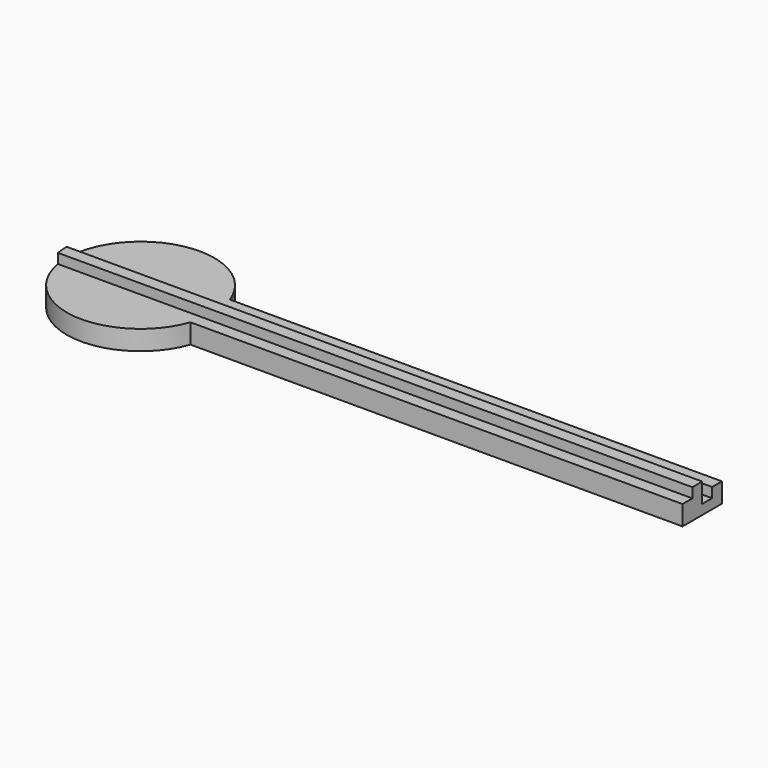
from build123d import *

# Parameters (mm, degrees)
F1_DEPTH = 2
F2_DEPTH = 3
F3_DEPTH = 1


with BuildPart() as f1:
    # F0 (on Top) → F1 (new body)
    with BuildSketch(Plane.XY):
        with BuildLine():
            ThreePointArc((-59.7277300679, 28.8946466617), (-59.8627935828, 28.2626599001), (-60.0517619849, 27.6446466617))
            Line((-60.0517619849, 27.6446466617), (-10.0517619849, 27.6446466617))
            Line((-10.0517619849, 27.6446466617), (-10.0517619849, 28.8946466617))
            Line((-10.0517619849, 28.8946466617), (-59.7277300679, 28.8946466617))
        make_face()
        with BuildLine():
            ThreePointArc((-74.5179295257, 28.8946466617), (-67.7684877332, 22.6724899563), (-60.0517619849, 27.6446466617))
            ThreePointArc((-60.0517619849, 27.6446466617), (-59.8627935828, 28.2626599001), (-59.7277300679, 28.8946466617))
            Line((-59.7277300679, 28.8946466617), (-74.5179295257, 28.8946466617))
        make_face()
        with BuildLine():
            ThreePointArc((-74.6228297968, 30.1446466617), (-74.5965587177, 29.5174497096), (-74.5179295257, 28.8946466617))
            Line((-74.5179295257, 28.8946466617), (-59.7277300679, 28.8946466617))
            ThreePointArc((-59.7277300679, 28.8946466617), (-59.6491008759, 29.5174497096), (-59.6228297968, 30.1446466617))
            Line((-59.6228297968, 30.1446466617), (-74.6228297968, 30.1446466617))
        make_face()
    extrude(amount=F1_DEPTH)

    # F0 (on Top) → F2 (join)
    with BuildSketch(Plane.XY):
        with BuildLine():
            ThreePointArc((-74.6228297968, 30.1446466617), (-74.5965587177, 29.5174497096), (-74.5179295257, 28.8946466617))
            Line((-74.5179295257, 28.8946466617), (-59.7277300679, 28.8946466617))
            ThreePointArc((-59.7277300679, 28.8946466617), (-59.6491008759, 29.5174497096), (-59.6228297968, 30.1446466617))
            Line((-59.6228297968, 30.1446466617), (-74.6228297968, 30.1446466617))
        make_face()
        with BuildLine():
            ThreePointArc((-59.6228297968, 30.1446466617), (-59.6491008759, 29.5174497096), (-59.7277300679, 28.8946466617))
            Line((-59.7277300679, 28.8946466617), (-10.0517619849, 28.8946466617))
            Line((-10.0517619849, 28.8946466617), (-10.0517619849, 30.1446466617))
            Line((-10.0517619849, 30.1446466617), (-59.6228297968, 30.1446466617))
        make_face()
    extrude(amount=F2_DEPTH)



with BuildPart() as f1b:
    # F0 (on Top) → F1, piece 2 (new body)
    with BuildSketch(Plane.XY):
        with BuildLine():
            ThreePointArc((-60.0517619849, 32.6446466617), (-67.7684877332, 37.616803367), (-74.5179295257, 31.3946466617))
            Line((-74.5179295257, 31.3946466617), (-59.7277300679, 31.3946466617))
            ThreePointArc((-59.7277300679, 31.3946466617), (-59.8627935828, 32.0266334232), (-60.0517619849, 32.6446466617))
        make_face()
        with BuildLine():
            ThreePointArc((-60.0517619849, 32.6446466617), (-59.8627935828, 32.0266334232), (-59.7277300679, 31.3946466617))
            Line((-59.7277300679, 31.3946466617), (-10.0517619849, 31.3946466617))
            Line((-10.0517619849, 31.3946466617), (-10.0517619849, 32.6446466617))
            Line((-10.0517619849, 32.6446466617), (-60.0517619849, 32.6446466617))
        make_face()
    extrude(amount=F1_DEPTH)


with BuildPart() as f1_1:
    add(f1.part)

    add(f1b.part)  # F3 merges F1b
    # F0 (on Top) → F3 (join)
    with BuildSketch(Plane.XY):
        with BuildLine():
            ThreePointArc((-74.6228297968, 30.1446466617), (-74.5965587177, 29.5174497096), (-74.5179295257, 28.8946466617))
            Line((-74.5179295257, 28.8946466617), (-59.7277300679, 28.8946466617))
            ThreePointArc((-59.7277300679, 28.8946466617), (-59.6491008759, 29.5174497096), (-59.6228297968, 30.1446466617))
            Line((-59.6228297968, 30.1446466617), (-74.6228297968, 30.1446466617))
        make_face()
        with BuildLine():
            ThreePointArc((-74.5179295257, 31.3946466617), (-74.5965587177, 30.7718436138), (-74.6228297968, 30.1446466617))
            Line((-74.6228297968, 30.1446466617), (-59.6228297968, 30.1446466617))
            ThreePointArc((-59.6228297968, 30.1446466617), (-59.6491008759, 30.7718436138), (-59.7277300679, 31.3946466617))
            Line((-59.7277300679, 31.3946466617), (-74.5179295257, 31.3946466617))
        make_face()
        with BuildLine():
            ThreePointArc((-59.7277300679, 31.3946466617), (-59.6491008759, 30.7718436138), (-59.6228297968, 30.1446466617))
            Line((-59.6228297968, 30.1446466617), (-10.0517619849, 30.1446466617))
            Line((-10.0517619849, 30.1446466617), (-10.0517619849, 31.3946466617))
            Line((-10.0517619849, 31.3946466617), (-59.7277300679, 31.3946466617))
        make_face()
    extrude(amount=F3_DEPTH)


solid = f1_1.part
